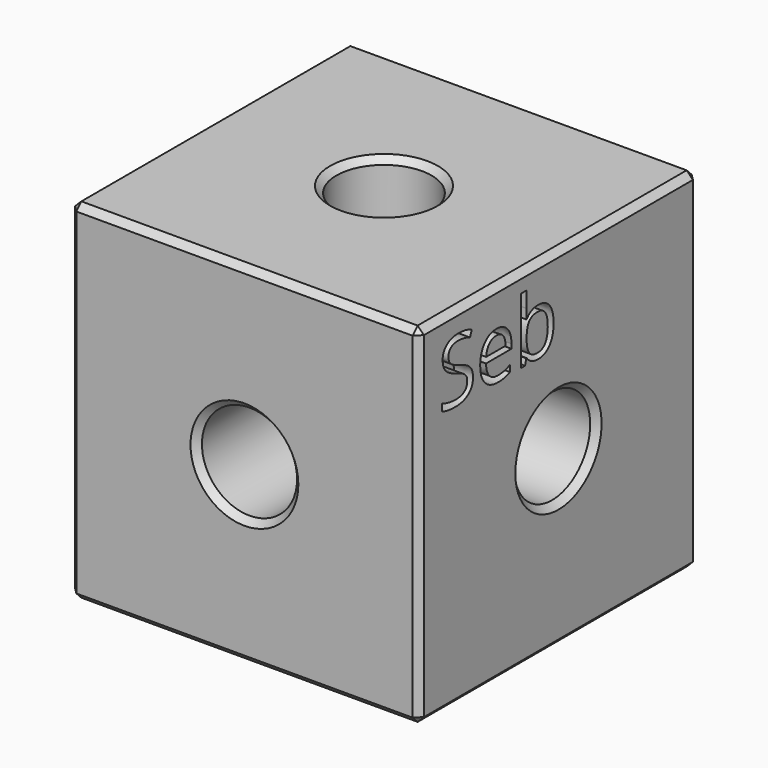
from build123d import *

# Parameters (mm, degrees)
F0_W         = 55
F0_H         = 55
F1_DEPTH     = 55
F3_D         = 15
F5_D         = 15
F7_D         = 15
F8_SIZE      = 1
F4_TEXT_SIZE = 13.60727
F9_DEPTH     = 3


# Not quite as in the source:
# - Text() gives the source's letters only with a copy of the font that has no kerning and outlines rounded to 1/6400 em; it was checked with that copy


with BuildPart() as f1:
    # F0 (on Top) → F1 (new body)
    with BuildSketch(Plane.XY):
        with Locations((-3.295775, -48.067693)):
            Rectangle(F0_W, F0_H)
    extrude(amount=F1_DEPTH)

    # F3 (through all)
    with Locations(Plane.XY.offset(55)):
        with Locations((-3.295775, -48.067693)):
            Hole(F3_D / 2)

    # F5 (through all)
    with Locations(Plane.YZ.offset(24.204225)):
        with Locations((-48.067693, 27.5)):
            Hole(F5_D / 2)

    # F7 (through all)
    with Locations(Plane(origin=(0, -20.567693, 0), x_dir=(-1, 0, 0), z_dir=(0, 1, 0))):
        with Locations((3.295775, 27.5)):
            Hole(F7_D / 2)

    # F8
    f8_edges = [f1.edges().sort_by_distance(p)[0] for p in [
        (24.204225, -48.067693, 55),
        (-3.295775, -75.567693, 55),
        (-3.295775, -20.567693, 55),
        (-30.795775, -48.067693, 55),
        (-10.795775, -48.067693, 55),
        (-30.795775, -75.567693, 27.5),
        (-3.295775, -75.567693, 0),
        (24.204225, -75.567693, 27.5),
        (4.204225, -75.567693, 27.5),
        (24.204225, -48.067693, 0),
        (24.204225, -20.567693, 27.5),
        (24.204225, -55.567693, 27.5),
        (-3.295775, -20.567693, 0),
        (-30.795775, -20.567693, 27.5),
        (4.204225, -20.567693, 27.5),
        (-30.795775, -48.067693, 0),
        (-30.795775, -55.567693, 27.5),
        (-10.795775, -48.067693, 0),
    ]]
    chamfer(f8_edges, length=F8_SIZE)

    # F4 (on face) → F9 (cut)
    with BuildSketch(Plane.YZ.offset(24.204225)):
        with Locations((-71.718391, 41.649595)):
            Text('Seb', F4_TEXT_SIZE, font='Open Sans', text_align=(TextAlign.LEFT, TextAlign.BOTTOM))
    extrude(amount=-F9_DEPTH, mode=Mode.SUBTRACT)


solid = f1.part
